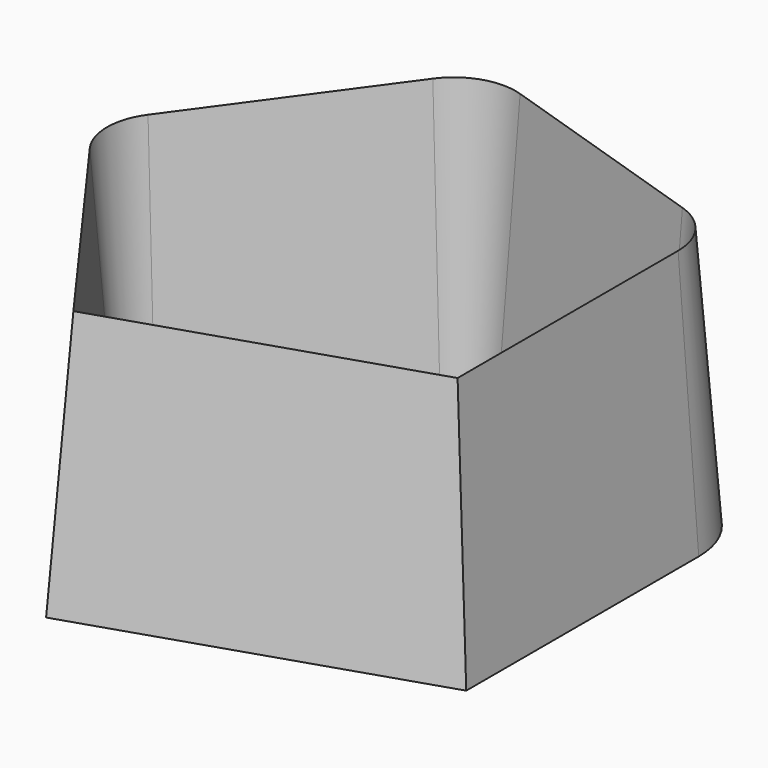
from build123d import *

# Parameters (mm, degrees)
F1_DEPTH = 85.344
F1_TAPER = 4.5


with BuildPart() as f1:
    # F0 (on Top) → F1 (new body)
    with BuildSketch(Plane.XY):
        with BuildLine():
            Line((37.095547, -26.951492), (37.095547, 17.724402))
            ThreePointArc((37.095547, 17.724402), (34.670063, 25.189275), (28.320063, 29.80282))
            Line((28.320063, 29.80282), (-5.393754, 40.757103))
            ThreePointArc((-5.393754, 40.757103), (-13.242786, 40.757103), (-19.592786, 36.143558))
            Line((-19.592786, 36.143558), (-40.42907, 7.464873))
            ThreePointArc((-40.42907, 7.464873), (-42.854554, 0), (-40.42907, -7.464873))
            Line((-40.42907, -7.464873), (-14.169238, -43.608431))
            Line((-14.169238, -43.608431), (37.095547, -26.951492))
        make_face()
        with BuildLine():
            ThreePointArc((-35.291813, -3.732437), (-36.504555, 0), (-35.291813, 3.732437))
            Line((-35.291813, 3.732437), (-14.455529, 32.411122))
            ThreePointArc((-14.455529, 32.411122), (-11.280528, 34.717895), (-7.356011, 34.717895))
            Line((-7.356011, 34.717895), (26.357805, 23.763612))
            ThreePointArc((26.357805, 23.763612), (29.532806, 21.456839), (30.745548, 17.724402))
            Line((30.745548, 17.724402), (30.745548, -22.337948))
            Line((30.745548, -22.337948), (-11.743754, -36.14356))
            Line((-11.743754, -36.14356), (-35.291813, -3.732437))
        make_face(mode=Mode.SUBTRACT)
    extrude(amount=F1_DEPTH, taper=F1_TAPER)


solid = f1.part
